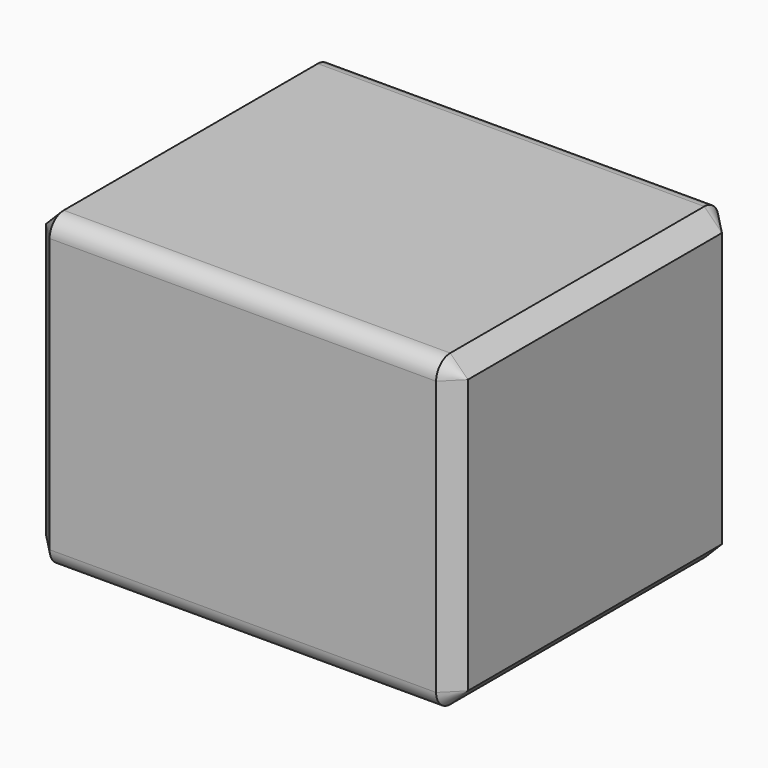
from build123d import *

# Parameters (mm, degrees)
F0_W     = 121.4544754475
F0_H     = 89.0452750027
F1_DEPTH = 101.6
F2_R     = 5.08
F3_SIZE  = 5.07999


# Not quite as in the source:
# - a fillet or chamfer is up to 0.001 mm smaller than in the source, because OpenCascade refuses the exact size


with BuildPart() as f1:
    # F0 (on Front) → F1 (new body)
    with BuildSketch(Plane.XZ):
        with Locations((-0.7558902726, 0.5788286217)):
            Rectangle(F0_W, F0_H)
    extrude(amount=F1_DEPTH)

    # F2
    f2_edges = [f1.edges().sort_by_distance(p)[0] for p in [
        (-0.75589, 0, 45.101466),
        (-0.75589, -101.6, 45.101466),
        (-0.75589, 0, -43.943809),
        (-0.75589, -101.6, -43.943809),
    ]]
    fillet(f2_edges, radius=F2_R)

    # F3 (size 5.08 in the source; OpenCascade refuses exactly that, so slightly less here)
    f3_edges = [f1.edges().sort_by_distance(p)[0] for p in [
        (59.971347, -50.8, -43.943809),
        (-61.483128, -50.8, -43.943809),
        (59.971347, -50.8, 45.101466),
        (-61.483128, -50.8, 45.101466),
    ]]
    chamfer(f3_edges, length=F3_SIZE)


solid = f1.part
